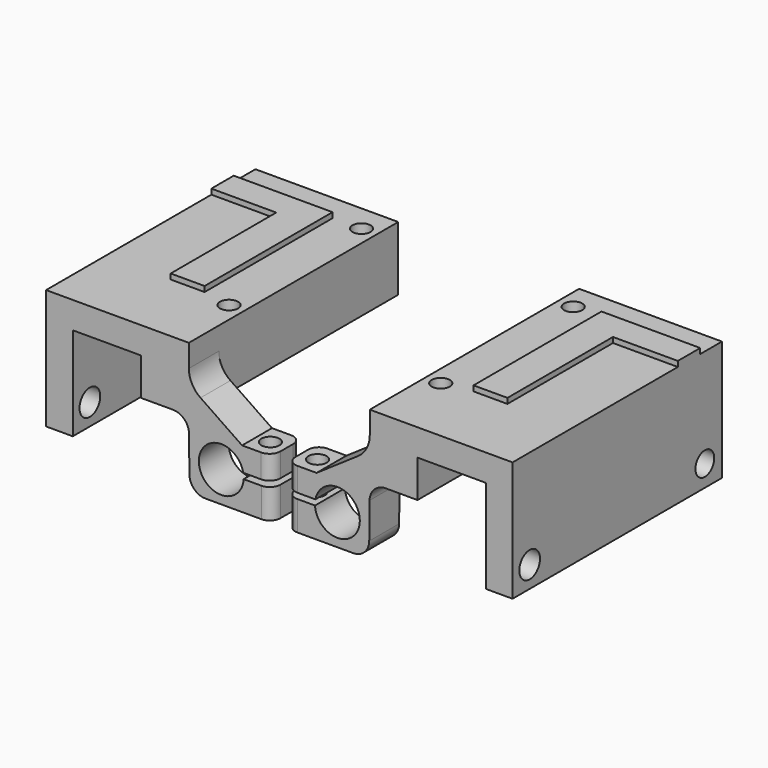
from build123d import *

# Parameters (mm, degrees)
F1_DEPTH      = 7
F2_DEPTH      = 42
F3_R          = 1.7
F3_R_2        = 11
F4_DEPTH      = 12.001
F5_R          = 4.2
F6_DEPTH      = 10
F7_DEPTH      = 12.001
F8_R          = 1.4
F9_DEPTH      = 10.9920075553
F8_R_2        = 1.7
F10_DEPTH     = 4.4348209087
F11_R         = 5
F12_R         = 3
F13_R         = 3
F14_R         = 2
F15_R         = 2.2
F15_R_2       = 2.4255023423
F16_DEPTH     = 6
F17_TEXT_SIZE = 41.9437823343
F18_DEPTH     = 1


# Not quite as in the source:
# - a feature names something its author has since deleted; it is built from what else it names
# - Text() gives the source's letters only with a copy of the font that has no kerning and outlines rounded to 1/6400 em; it was checked with that copy


with BuildPart() as f1:
    # F0 (on Front) → F1 (new body)
    with BuildSketch(Plane.XZ):
        Polygon((-18.6721007523, 29.8099789735), (-18.6721007523, 7.3259699669), (-13.6721007523, 7.3259699669), (-13.6721007523, 24.8099789735), (-0.8721007523, 24.8099789735), (-0.8721007523, 17.8099789735), (8.0637966118, 17.8099789735), (8.0637966118, 22.9406704692), (8.0637966118, 29.8099789735), align=None)
        Polygon((18.0301751077, 16.1394868046), (8.0637966118, 22.9406704692), (8.0637966118, 17.8099789735), (8.1940201178, 5.1484792493), (23.6186601057, 5.1484792493), (23.6186601057, 10.6682249423), (16.2860510706, 10.6682249423), (16.2860510706, 11.7046658959), (23.5896428882, 11.7046658959), (23.5896428882, 16.1394868046), align=None)
    extrude(amount=F1_DEPTH)

    # F0 (on Front) → F2 (join)
    with BuildSketch(Plane.XZ):
        Polygon((-18.6721007523, 29.8099789735), (-18.6721007523, 7.3259699669), (-13.6721007523, 7.3259699669), (-13.6721007523, 24.8099789735), (-0.8721007523, 24.8099789735), (-0.8721007523, 17.8099789735), (8.0637966118, 17.8099789735), (8.0637966118, 22.9406704692), (8.0637966118, 29.8099789735), align=None)
    extrude(amount=-F2_DEPTH)

    # F3 (on face) → F4 (cut, through all)
    with BuildSketch(Plane(origin=(0, 0, 17.8099789735), x_dir=(1, 0, 0), z_dir=(0, 0, -1))):
        with Locations((5.1850692477, -6)):
            Circle(F3_R)
        with Locations((5.1850692477, -37)):
            Circle(F3_R)
        with Locations((20.6850692477, -21.5)):
            Circle(F3_R_2)
    extrude(amount=-F4_DEPTH, mode=Mode.SUBTRACT)

    # F5 (on face) → F6 (cut)
    with BuildSketch(Plane.XZ.offset(7)):
        with Locations((14.1278992477, 10.8989789735)):
            Circle(F5_R)
    extrude(amount=-F6_DEPTH, mode=Mode.SUBTRACT)

    # F3 (on face) → F7 (cut, through all)
    with BuildSketch(Plane(origin=(0, 0, 17.8099789735), x_dir=(1, 0, 0), z_dir=(0, 0, -1))):
        with Locations((5.1850692477, -6)):
            Circle(F3_R)
        with Locations((5.1850692477, -37)):
            Circle(F3_R)
        with Locations((20.6850692477, -21.5)):
            Circle(F3_R_2)
    extrude(amount=-F7_DEPTH, mode=Mode.SUBTRACT)

    # F8 (on face) → F9 (cut, through all)
    with BuildSketch(Plane.XY.offset(16.1394868046)):
        with Locations((20.5896428882, -3.5767070949)):
            Circle(F8_R)
    extrude(amount=-F9_DEPTH, mode=Mode.SUBTRACT)

    # F8 (on face) → F10 (cut, through all)
    with BuildSketch(Plane.XY.offset(16.1394868046)):
        with Locations((20.5896428882, -3.5767070949)):
            Circle(F8_R_2)
        with Locations((20.5896428882, -3.5767070949)):
            Circle(F8_R, mode=Mode.SUBTRACT)
    extrude(amount=-F10_DEPTH, mode=Mode.SUBTRACT)

    # F11
    f11_edges = [f1.edges().sort_by_distance(p)[0] for p in [
        (8.063797, -3.5, 22.94067),
    ]]
    fillet(f11_edges, radius=F11_R)

    # F12
    f12_edges = [f1.edges().sort_by_distance(p)[0] for p in [
        (8.063797, -3.5, 17.809979),
    ]]
    fillet(f12_edges, radius=F12_R)

    # F13
    f13_edges = [f1.edges().sort_by_distance(p)[0] for p in [
        (8.19402, -3.5, 5.148479),
    ]]
    fillet(f13_edges, radius=F13_R)

    # F14
    f14_edges = [f1.edges().sort_by_distance(p)[0] for p in [
        (23.589643, -7, 13.922076),
        (23.61866, -7, 7.908352),
        (23.589643, 0, 13.922076),
        (23.61866, 0, 7.908352),
    ]]
    fillet(f14_edges, radius=F14_R)

    # F15 (on face) → F16 (cut)
    with BuildSketch(Plane(origin=(-18.6721007523, 0, 0), x_dir=(0, -1, 0), z_dir=(-1, 0, 0))):
        with Locations((-38, 11.3259699669)):
            Circle(F15_R)
        with Locations((3, 11.3259699669)):
            Circle(F15_R_2)
    extrude(amount=-F16_DEPTH, mode=Mode.SUBTRACT)

    # F17 (on face) → F18 (join)
    with BuildSketch(Plane.XY.offset(29.8099789735)):
        with Locations(Location((3.5908724648, 36.9253193088), (0, 0, 180))):
            Text('L', F17_TEXT_SIZE, font='Open Sans', font_style=FontStyle.BOLD, text_align=(TextAlign.LEFT, TextAlign.BOTTOM))
    extrude(amount=F18_DEPTH)


with BuildPart() as f19_1:
    # F19: instance of F1
    add(f1.part.mirror(Plane.YZ))


with BuildPart() as f19_1_1:
    # F20: moved
    add(f19_1.part.moved(Location((50, 0, 0))))


solid = Compound([f1.part, f19_1_1.part])
